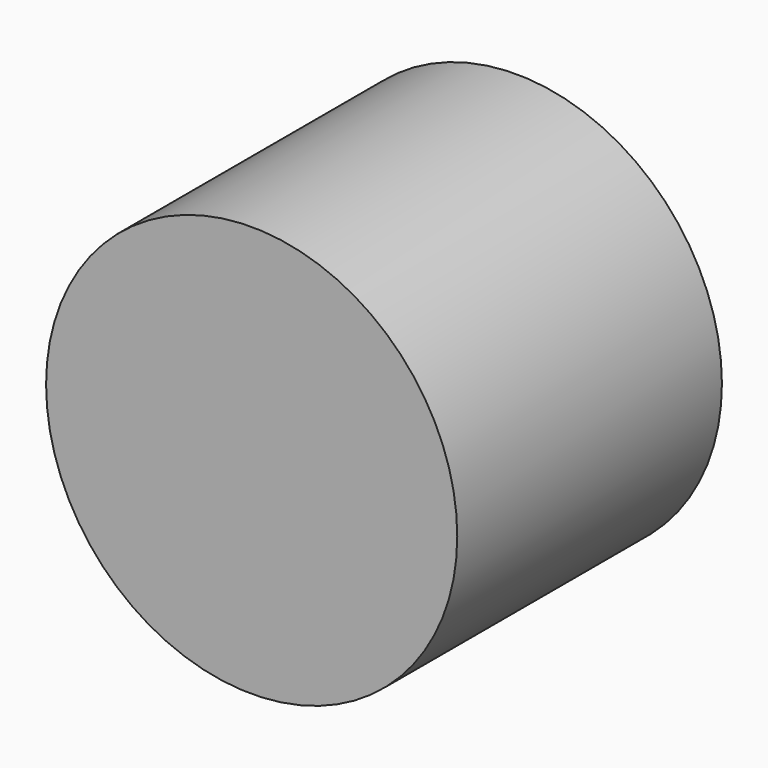
from build123d import *

# Parameters (mm, degrees)
F1_R     = 1.5784229559
F2_DEPTH = 2.54


# Not quite as in the source:
# - the program builds the solid bodies; features that only make, move or delete a surface that nothing else refers to are left out


with BuildPart() as f2:
    # F1 (on Front) → F2 (new body)
    with BuildSketch(Plane.XZ):
        with Locations((-13.8561800122, 64.5654797554)):
            Circle(F1_R)
    extrude(amount=F2_DEPTH)


solid = f2.part
